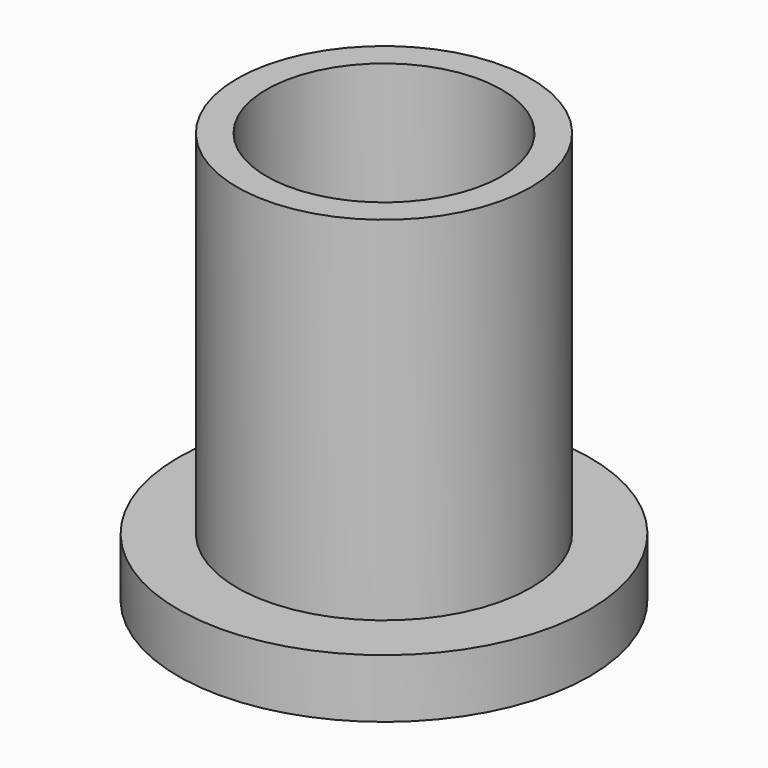
from build123d import *

# Parameters (mm, degrees)
F0_R     = 17.5
F1_DEPTH = 5
F2_R     = 12.5
F3_DEPTH = 30
F4_T     = 2.5


# Not quite as in the source:
# - a shell that OpenCascade refuses in one call is made with other operations: the cavity is built on its own and cut out


with BuildPart() as f1:
    # F0 (on Top) → F1 (new body)
    with BuildSketch(Plane.XY):
        Circle(F0_R)
    extrude(amount=F1_DEPTH)

    # F2 (on face) → F3 (join)
    with BuildSketch(Plane.XY.offset(5)):
        Circle(F2_R)
    extrude(amount=F3_DEPTH)

    # F4: shell of thickness 2.5, made by hand


with BuildPart() as f4_core1:
    # F4_t2: copy of F1
    add(f1.part)

    # the walls: a layer under each face that stays
    f4_faces = [f4_core1.faces().sort_by_distance(p)[0] for p in [
        (-17.5, 0, 2.5),
        (0, 0, 0),
        (-11.6666666667, -11.6666666667, 5),
        (-12.5, 0, 20),
    ]]
    thicken(f4_faces, amount=-F4_T, mode=Mode.SUBTRACT)

    # F4_s3 → F4_t4 (revolve, cut)
    with BuildSketch(Plane.XZ):
        Polygon((12.525, 5.025), (12.5, 2.5), (10, 2.5), (10, 5), align=None)
    revolve(axis=Axis((0, 0, 5), (0, 0, 1)), mode=Mode.SUBTRACT)


with BuildPart() as f1_1:
    add(f1.part)

    # what is left inside the walls is the cavity
    f4_cavity = [f4_core1.part.solids().sort_by_distance(p)[0] for p in [
        (-9.975, 0, 13.333333),
    ]]
    add(f4_cavity, mode=Mode.SUBTRACT)


solid = f1_1.part
